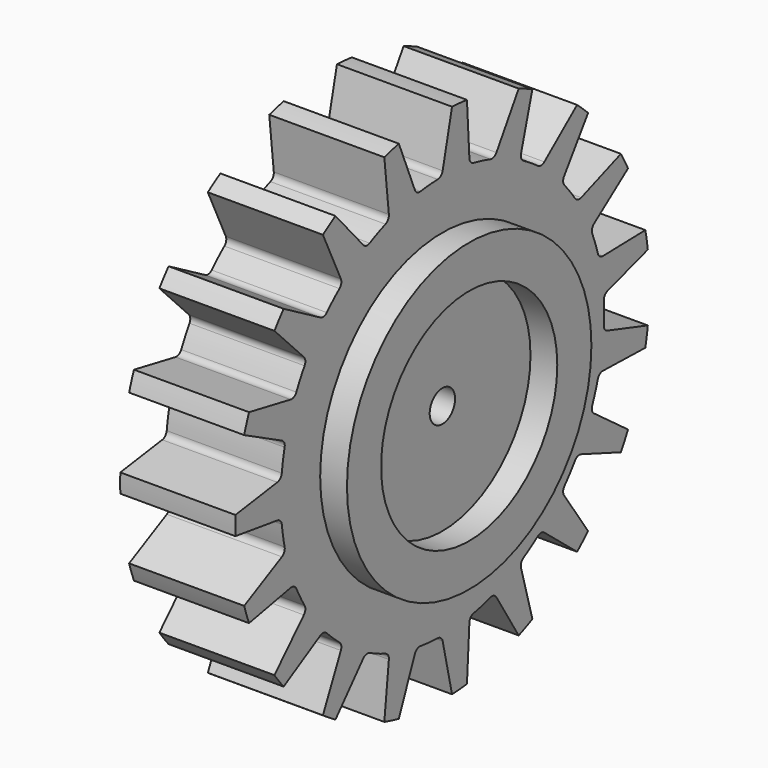
from build123d import *

# Parameters (mm, degrees)
F3_DEPTH        = 76.2
F3_COPIES_COUNT = 19
F4_R            = 1.27


# Not quite as in the source:
# - a feature of the source that left no trace in its solid (it failed there, or was rolled back) is left out
# - a pattern or mirror of a feature is missing from the dataset's text; its kind, count and spacing are read off the source's solid


with BuildPart() as f1:
    # F0 (on Top) → F1 (revolve)
    with BuildSketch(Plane.XY):
        Polygon((-11.7041012272, 21.2976261973), (-11.7041012272, 3.0699281488), (10.5528766289, 3.0699281488), (10.5528766289, 21.2976261973), (15.7333817333, 21.2976261973), (15.7333817333, 29.5480582863), (10.5528766289, 29.5480582863), (10.5528766289, 50.0781983137), (-11.7041012272, 50.0781983137), (-11.7041012272, 29.5480582863), (-17.0764755458, 29.5480582863), (-17.0764755458, 21.2976261973), align=None)
    revolve(axis=Axis((-9.8813325167, 0, 0), (1, 0, 0)))

    # F2 (on Right) → F3 (cut, symmetric)
    with BuildSketch(Plane.YZ):
        with BuildLine():
            ThreePointArc((49.8863309622, -6.5235970542), (50.311065735, 0), (49.8863309622, 6.5235970542))
            Line((49.8863309622, 6.5235970542), (38.9497131109, 3.0699283816))
            ThreePointArc((38.9497131109, 3.0699283816), (39.0705082088, 0), (38.9497131109, -3.0699283816))
            Line((38.9497131109, -3.0699283816), (49.8863309622, -6.5235970542))
        make_face()
    f3 = extrude(amount=F3_DEPTH, both=True, mode=Mode.SUBTRACT)

    # F3_copies: F3 ×19 about axis
    f3_copies_axis = Axis((0, 0, 0), (1, 0, 0))
    for i in range(1, F3_COPIES_COUNT):
        add(f3.rotate(f3_copies_axis, i * 360 / F3_COPIES_COUNT), mode=Mode.SUBTRACT)

    # F4
    f4_edges = [f1.edges().sort_by_distance(p)[0] for p in [
        (-0.575612, 38.949713, 3.069928),
        (-0.575612, 38.949713, -3.069928),
        (-0.575612, 37.836114, -9.74336),
        (-0.575612, 35.842506, -15.550542),
        (-0.575612, 32.622385, -21.500804),
        (-0.575612, 28.851207, -26.346014),
        (-0.575612, 23.873515, -30.928302),
        (-0.575612, 18.733433, -34.286486),
        (-0.575612, 12.537579, -37.004239),
        (-0.575612, 6.5856, -38.511485),
        (-0.575612, -0.156999, -39.070193),
        (-0.575612, -6.275885, -38.563167),
        (-0.575612, -12.834563, -36.902285),
        (-0.575612, -18.45728, -34.435932),
        (-0.575612, -24.121303, -30.735441),
        (-0.575612, -28.638543, -26.577029),
        (-0.575612, -32.794126, -21.237936),
        (-0.575612, -35.716375, -15.838093),
        (-0.575612, -37.913196, -9.438971),
        (-0.575612, -38.923783, -3.382854),
        (-0.575612, -38.923783, 3.382854),
        (-0.575612, -37.913196, 9.438971),
        (-0.575612, -35.716375, 15.838093),
        (-0.575612, -32.794126, 21.237936),
        (-0.575612, -28.638543, 26.577029),
        (-0.575612, -24.121303, 30.735441),
        (-0.575612, -18.45728, 34.435932),
        (-0.575612, -12.834563, 36.902285),
        (-0.575612, -6.275885, 38.563167),
        (-0.575612, -0.156999, 39.070193),
        (-0.575612, 6.5856, 38.511485),
        (-0.575612, 12.537579, 37.004239),
        (-0.575612, 18.733433, 34.286486),
        (-0.575612, 23.873515, 30.928302),
        (-0.575612, 28.851207, 26.346014),
        (-0.575612, 32.622385, 21.500804),
        (-0.575612, 35.842506, 15.550542),
        (-0.575612, 37.836114, 9.74336),
    ]]
    fillet(f4_edges, radius=F4_R)


solid = f1.part
